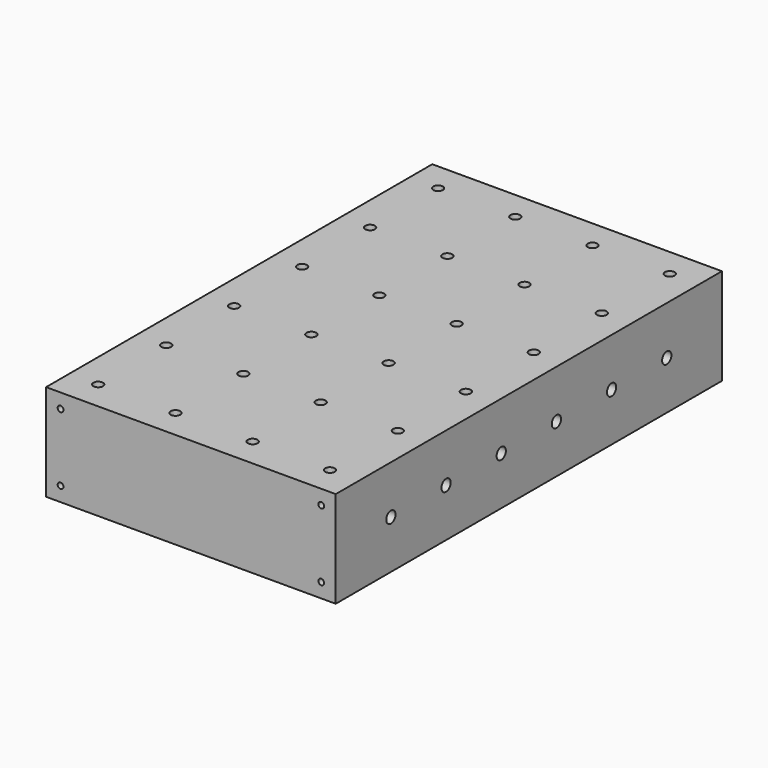
from build123d import *

# Parameters (mm, degrees)
F0_W          = 300
F0_H          = 500
F1_DEPTH      = 100
F4_DEPTH      = 225
F4_DEPTH_BACK = 225
F5_DEPTH      = 225
F5_DEPTH_BACK = 225
F2_R          = 7.5
F6_DEPTH      = 25
F7_R          = 6
F8_DEPTH      = 25
F9_R          = 6
F10_DEPTH     = 25
F11_R         = 3
F12_DEPTH     = 10
F13_R         = 3
F14_DEPTH     = 10
F15_R         = 5
F16_DEPTH     = 15


# Not quite as in the source:
# - a feature of the source that left no trace in its solid (it failed there, or was rolled back) is left out


with BuildPart() as f1:
    # F0 (on Top) → F1 (new body)
    with BuildSketch(Plane.XY):
        Rectangle(F0_W, F0_H)
    extrude(amount=F1_DEPTH)

    # F3 (on Front) → F4 (cut, two sides)
    with BuildSketch(Plane.XZ) as f4_sk:
        Polygon((150, 17.5), (150, 82.5), (120, 82.5), (120, 67.5), (140, 67.5), (140, 32.5), (120, 32.5), (120, 17.5), align=None)
        Polygon((-120, 82.5), (-150, 82.5), (-150, 17.5), (-120, 17.5), (-120, 32.5), (-140, 32.5), (-140, 67.5), (-120, 67.5), align=None)
    extrude(amount=-F4_DEPTH, mode=Mode.SUBTRACT)
    extrude(f4_sk.sketch, amount=F4_DEPTH_BACK, mode=Mode.SUBTRACT)

    # F3 (on Front) → F5 (join, two sides)
    with BuildSketch(Plane.XZ) as f5_sk:
        Polygon((150, 17.5), (150, 82.5), (120, 82.5), (120, 67.5), (140, 67.5), (140, 32.5), (120, 32.5), (120, 17.5), align=None)
        Polygon((-120, 82.5), (-150, 82.5), (-150, 17.5), (-120, 17.5), (-120, 32.5), (-140, 32.5), (-140, 67.5), (-120, 67.5), align=None)
    extrude(amount=F5_DEPTH)
    extrude(f5_sk.sketch, amount=-F5_DEPTH_BACK)

    # F2 (on face) → F6 (cut)
    with BuildSketch(Plane(origin=(0, 0, 0), x_dir=(1, 0, 0), z_dir=(0, 0, -1))):
        with Locations((-100, 200)):
            Circle(F2_R)
        with Locations((100, 200)):
            Circle(F2_R)
        with Locations((100, -200)):
            Circle(F2_R)
        with Locations((-100, -200)):
            Circle(F2_R)
    extrude(amount=-F6_DEPTH, mode=Mode.SUBTRACT)

    # F7 (on face) → F8 (cut)
    with BuildSketch(Plane(origin=(-150, 0, 0), x_dir=(0, -1, 0), z_dir=(-1, 0, 0))):
        with Locations((-178.5714285714, 50)):
            Circle(F7_R)
        with Locations((-107.1428571429, 50)):
            Circle(F7_R)
        with Locations((-35.7142857143, 50)):
            Circle(F7_R)
        with Locations((35.7142857143, 50)):
            Circle(F7_R)
        with Locations((107.1428571429, 50)):
            Circle(F7_R)
        with Locations((178.5714285714, 50)):
            Circle(F7_R)
    extrude(amount=-F8_DEPTH, mode=Mode.SUBTRACT)

    # F9 (on face) → F10 (cut)
    with BuildSketch(Plane.YZ.offset(150)):
        with Locations((-178.5714285714, 50)):
            Circle(F9_R)
        with Locations((-107.1428571429, 50)):
            Circle(F9_R)
        with Locations((-35.7142857143, 50)):
            Circle(F9_R)
        with Locations((35.7142857143, 50)):
            Circle(F9_R)
        with Locations((107.1428571429, 50)):
            Circle(F9_R)
        with Locations((178.5714285714, 50)):
            Circle(F9_R)
    extrude(amount=-F10_DEPTH, mode=Mode.SUBTRACT)

    # F11 (on face) → F12 (cut)
    with BuildSketch(Plane(origin=(0, 250, 0), x_dir=(-1, 0, 0), z_dir=(0, 1, 0))):
        with Locations((-135, 85)):
            Circle(F11_R)
        with Locations((-135, 15)):
            Circle(F11_R)
        with Locations((135, 15)):
            Circle(F11_R)
        with Locations((135, 85)):
            Circle(F11_R)
    extrude(amount=-F12_DEPTH, mode=Mode.SUBTRACT)

    # F13 (on face) → F14 (cut)
    with BuildSketch(Plane.XZ.offset(250)):
        with Locations((135, 85)):
            Circle(F13_R)
        with Locations((135, 15)):
            Circle(F13_R)
        with Locations((-135, 15)):
            Circle(F13_R)
        with Locations((-135, 85)):
            Circle(F13_R)
    extrude(amount=-F14_DEPTH, mode=Mode.SUBTRACT)

    # F15 (on face) → F16 (cut)
    with BuildSketch(Plane.XY.offset(100)):
        with Locations((120, 220)):
            Circle(F15_R)
        with Locations((120, 132)):
            Circle(F15_R)
        with Locations((120, 44)):
            Circle(F15_R)
        with Locations((120, -44)):
            Circle(F15_R)
        with Locations((120, -132)):
            Circle(F15_R)
        with Locations((120, -220)):
            Circle(F15_R)
        with Locations((40, 220)):
            Circle(F15_R)
        with Locations((40, 132)):
            Circle(F15_R)
        with Locations((40, 44)):
            Circle(F15_R)
        with Locations((40, -44)):
            Circle(F15_R)
        with Locations((40, -132)):
            Circle(F15_R)
        with Locations((40, -220)):
            Circle(F15_R)
        with Locations((-40, 220)):
            Circle(F15_R)
        with Locations((-40, 132)):
            Circle(F15_R)
        with Locations((-40, 44)):
            Circle(F15_R)
        with Locations((-40, -44)):
            Circle(F15_R)
        with Locations((-40, -132)):
            Circle(F15_R)
        with Locations((-40, -220)):
            Circle(F15_R)
        with Locations((-120, 220)):
            Circle(F15_R)
        with Locations((-120, 132)):
            Circle(F15_R)
        with Locations((-120, 44)):
            Circle(F15_R)
        with Locations((-120, -44)):
            Circle(F15_R)
        with Locations((-120, -132)):
            Circle(F15_R)
        with Locations((-120, -220)):
            Circle(F15_R)
    extrude(amount=-F16_DEPTH, mode=Mode.SUBTRACT)


solid = f1.part
